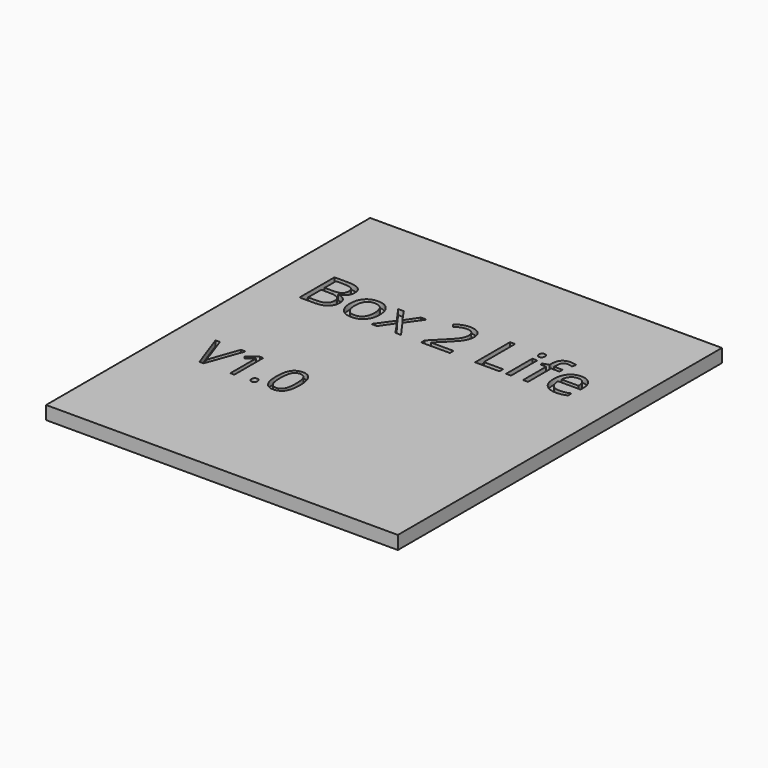
from build123d import *

# Parameters (mm, degrees)
F0_W           = 66
F0_H           = 76
F1_DEPTH       = 2.5
F2_TEXT_SIZE   = 11.4856856979
F2_TEXT_SIZE_2 = 9.5053963984
F3_DEPTH       = 1


# Not quite as in the source:
# - Text() gives the source's letters only with a copy of the font that has no kerning and outlines rounded to 1/6400 em; it was checked with that copy


with BuildPart() as f1:
    # F0 (on Top) → F1 (new body)
    with BuildSketch(Plane.XY):
        with Locations((33, 38)):
            Rectangle(F0_W, F0_H)
    extrude(amount=F1_DEPTH)

    # F2 (on face) → F3 (cut)
    with BuildSketch(Plane.XY.offset(2.5)):
        with Locations((6.5587246791, 49.8330034316)):
            Text('Box 2 Life', F2_TEXT_SIZE, font='Open Sans', text_align=(TextAlign.LEFT, TextAlign.BOTTOM))
        with Locations((6.5587246791, 24.7387569398)):
            Text('V1.0', F2_TEXT_SIZE_2, font='Open Sans', text_align=(TextAlign.LEFT, TextAlign.BOTTOM))
    extrude(amount=-F3_DEPTH, mode=Mode.SUBTRACT)


solid = f1.part
